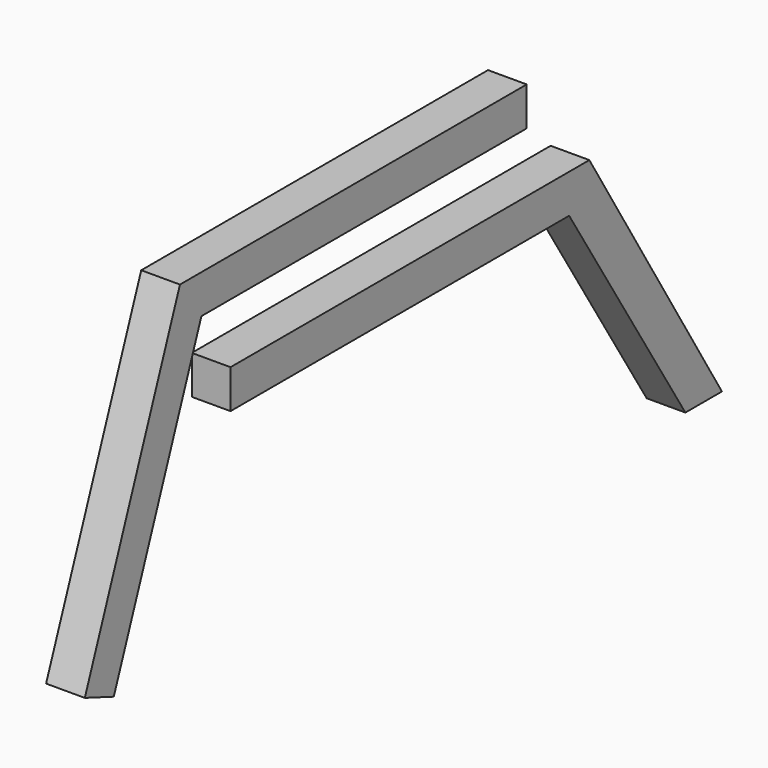
from build123d import *

# Parameters (mm, degrees)
F2_DEPTH = 20
F3_DEPTH = 20


with BuildPart() as f2:
    # F1 (on Right) → F2 (new body)
    with BuildSketch(Plane.YZ):
        Polygon((-151.5351831913, -75), (-95, 75), (-49.1520948708, 75), (-49.1520948708, 95), (-108.8353658587, 95), (-170.2500428688, -67.9463465316), align=None)
        Polygon((-49.1520948708, 95), (-49.1520948708, 75), (95, 75), (115, 75), (115, 95), (95, 95), align=None)
    extrude(amount=F2_DEPTH)


with BuildPart() as f3:
    # F0 (on Right) → F3 (new body)
    with BuildSketch(Plane.YZ):
        Polygon((217.7155762911, -95.8306404948), (241.000726819, -95.8306404948), (167.650522438, 24.1693595052), (142.3945370404, 24.1693595052), (217.4223265664, -95.8306404948), align=None)
        Polygon((142.3945370404, 24.1693595052), (167.650522438, 24.1693595052), (155.4254883744, 44.1693595052), (129.8899054527, 44.1693595052), align=None)
        Polygon((-76.201092194, 24.1693595052), (142.3945370404, 24.1693595052), (129.8899054527, 44.1693595052), (-76.201092194, 44.1693595052), align=None)
    extrude(amount=F3_DEPTH)


solid = Compound([f2.part, f3.part])
